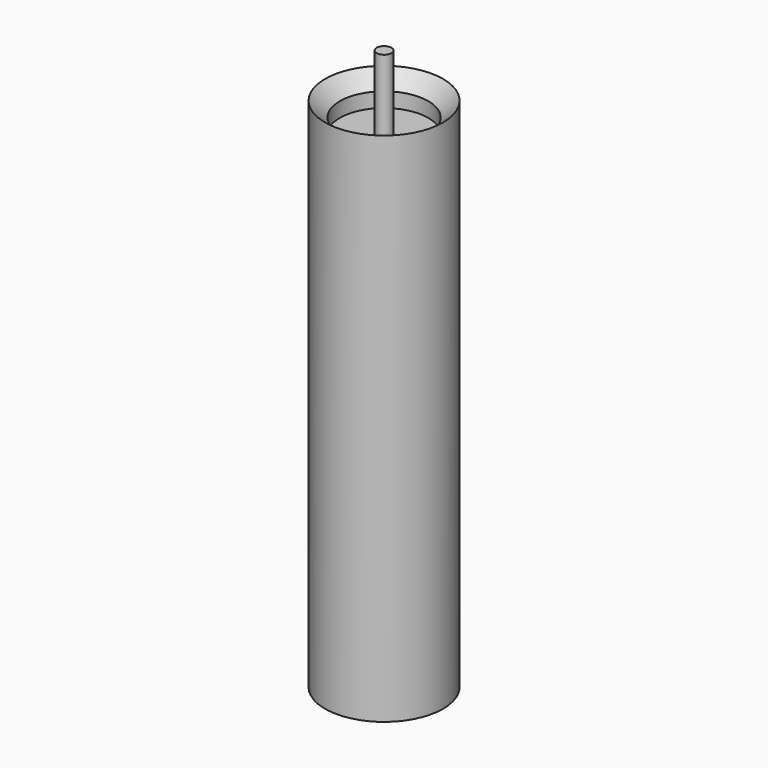
from build123d import *

# Parameters (mm, degrees)
F0_R     = 4
F0_R_2   = 3
F1_DEPTH = 20
F2_DEPTH = 15
F3_DEPTH = 13
F4_SIZE  = 0.99999
F5_R     = 0.5
F6_DEPTH = 5


# Not quite as in the source:
# - a fillet or chamfer is up to 0.001 mm smaller than in the source, because OpenCascade refuses the exact size


with BuildPart() as f1:
    # F0 (on Top) → F1 (new body)
    with BuildSketch(Plane.XY):
        Circle(F0_R)
        Circle(F0_R_2, mode=Mode.SUBTRACT)
    extrude(amount=-F1_DEPTH)

    # F0 (on Top) → F2 (join)
    with BuildSketch(Plane.XY):
        Circle(F0_R)
        Circle(F0_R_2, mode=Mode.SUBTRACT)
    extrude(amount=F2_DEPTH)

    # F0 (on Top) → F3 (join)
    with BuildSketch(Plane.XY):
        Circle(F0_R_2)
    extrude(amount=F3_DEPTH)

    # F4 (size 1 in the source; OpenCascade refuses exactly that, so slightly less here)
    f4_edges = [f1.edges().sort_by_distance(p)[0] for p in [
        (-3, 0, 15),
    ]]
    chamfer(f4_edges, length=F4_SIZE)

    # F5 (on face) → F6 (join)
    with BuildSketch(Plane.XY.offset(13)):
        Circle(F5_R)
    extrude(amount=F6_DEPTH)


solid = f1.part
